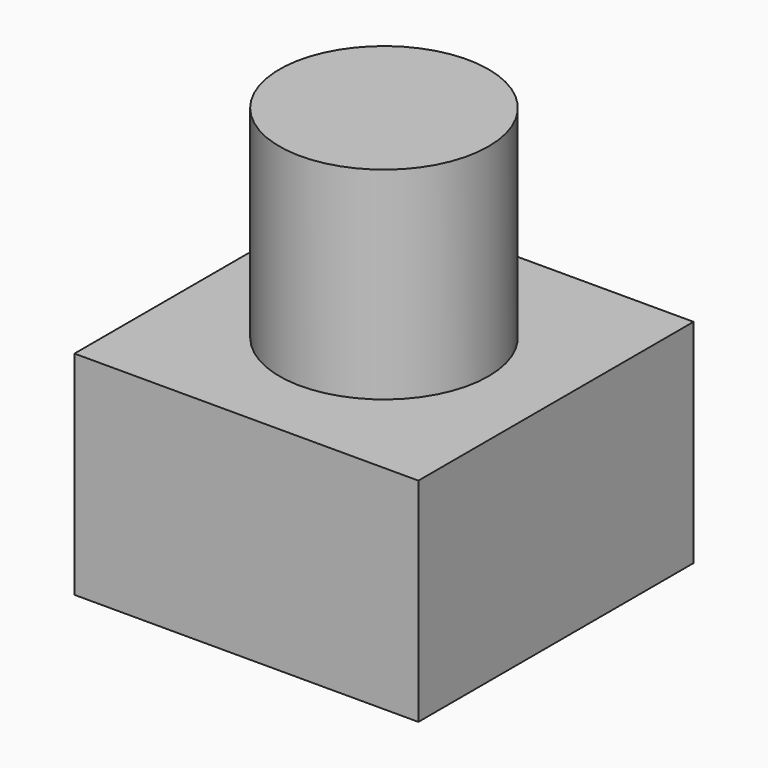
from build123d import *

# Parameters (mm, degrees)
F0_R     = 15.5
F1_DEPTH = 30
F2_W     = 51
F2_H     = 51
F3_DEPTH = 1
F4_W     = 51
F4_H     = 51
F4_W_2   = 31
F4_H_2   = 31
F5_DEPTH = 30.5


with BuildPart() as f1:
    # F0 (on Top) → F1 (new body)
    with BuildSketch(Plane.XY):
        Circle(F0_R)
    extrude(amount=F1_DEPTH)

    # F2 (on face) → F3 (join)
    with BuildSketch(Plane(origin=(0, 0, 0), x_dir=(1, 0, 0), z_dir=(0, 0, -1))):
        Rectangle(F2_W, F2_H)
        Polygon((15.5, 0), (15.5, -15.5), (0, -15.5), (-15.5, -15.5), (-15.5, 0), (-15.5, 15.5), (-6.64e-08, 15.5), (15.5, 15.5), align=None, mode=Mode.SUBTRACT)
        with BuildLine():
            Line((0, -15.5), (15.5, -15.5))
            Line((15.5, -15.5), (15.5, 0))
            ThreePointArc((15.5, 0), (10.9601551084, -10.9601551084), (0, -15.5))
        make_face()
        with BuildLine():
            Line((-15.5, -15.5), (0, -15.5))
            ThreePointArc((0, -15.5), (-10.9601551084, -10.9601551084), (-15.5, 0))
            Line((-15.5, 0), (-15.5, -15.5))
        make_face()
        with BuildLine():
            ThreePointArc((-15.5, 0), (-10.9601551084, -10.9601551084), (0, -15.5))
            ThreePointArc((0, -15.5), (10.9601551084, -10.9601551084), (15.5, 0))
            ThreePointArc((15.5, 0), (10.9601550849, 10.9601551319), (-6.64e-08, 15.5))
            ThreePointArc((-6.64e-08, 15.5), (-10.9601551319, 10.9601550849), (-15.5, 0))
        make_face()
        with BuildLine():
            ThreePointArc((-6.64e-08, 15.5), (10.9601550849, 10.9601551319), (15.5, 0))
            Line((15.5, 0), (15.5, 15.5))
            Line((15.5, 15.5), (-6.64e-08, 15.5))
        make_face()
        with BuildLine():
            Line((-15.5, 15.5), (-15.5, 0))
            ThreePointArc((-15.5, 0), (-10.9601551319, 10.9601550849), (-6.64e-08, 15.5))
            Line((-6.64e-08, 15.5), (-15.5, 15.5))
        make_face()
    extrude(amount=F3_DEPTH)

    # F4 (on face) → F5 (join)
    with BuildSketch(Plane(origin=(0, 0, -1), x_dir=(1, 0, 0), z_dir=(0, 0, -1))):
        Rectangle(F4_W, F4_H)
        Rectangle(F4_W_2, F4_H_2, mode=Mode.SUBTRACT)
    extrude(amount=F5_DEPTH)


solid = f1.part
